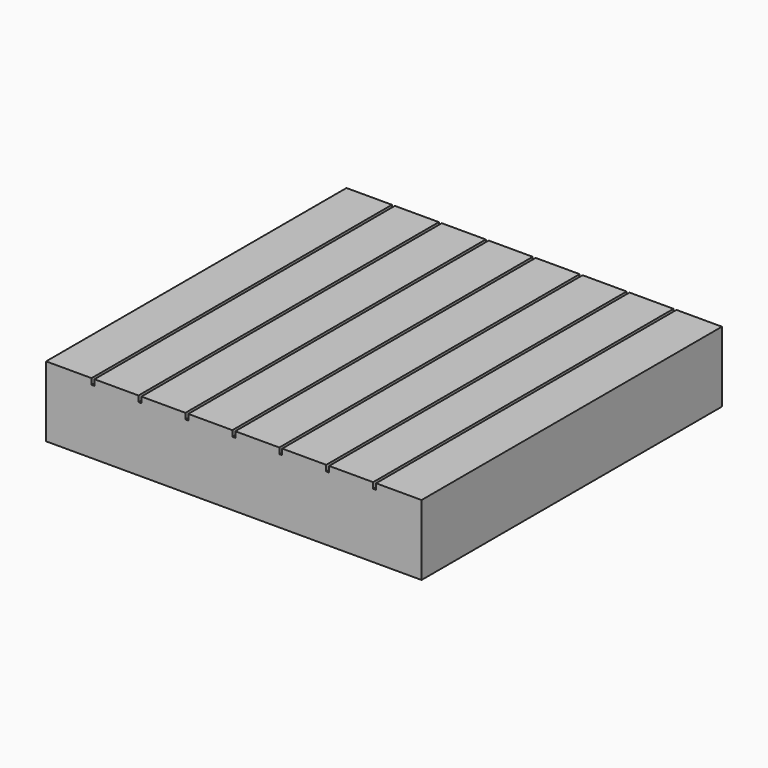
from build123d import *

# Parameters (mm, degrees)
F0_W     = 101.6
F0_H     = 101.6
F1_DEPTH = 19.05
F2_W     = 0.396875
F2_H     = 101.6
F3_DEPTH = 1.5875


# Not quite as in the source:
# - a length typed as a fraction of an inch, garbled in the dataset ("3 / 203.2 mm" for 3/8 in), is restored


with BuildPart() as f1:
    # F0 (on Top) → F1 (new body)
    with BuildSketch(Plane.XY):
        Rectangle(F0_W, F0_H)
    extrude(amount=F1_DEPTH)

    # F2 (on face) → F3 (cut)
    with BuildSketch(Plane.XY.offset(19.05)):
        with Locations((-38.2984375, 0)):
            Rectangle(F2_W, F2_H)
        with Locations((-37.9015625, 0)):
            Rectangle(F2_W, F2_H)
        with Locations((-25.5984375, 0)):
            Rectangle(F2_W, F2_H)
        with Locations((-25.2015625, 0)):
            Rectangle(F2_W, F2_H)
        with Locations((-12.8984375, 0)):
            Rectangle(F2_W, F2_H)
        with Locations((-12.5015625, 0)):
            Rectangle(F2_W, F2_H)
        with Locations((-0.1984375, 0)):
            Rectangle(F2_W, F2_H)
        with Locations((0.1984375, 0)):
            Rectangle(F2_W, F2_H)
        with Locations((12.5015625, 0)):
            Rectangle(F2_W, F2_H)
        with Locations((12.8984375, 0)):
            Rectangle(F2_W, F2_H)
        with Locations((25.2015625, 0)):
            Rectangle(F2_W, F2_H)
        with Locations((25.5984375, 0)):
            Rectangle(F2_W, F2_H)
        with Locations((37.9015625, 0)):
            Rectangle(F2_W, F2_H)
        with Locations((38.2984375, 0)):
            Rectangle(F2_W, F2_H)
    extrude(amount=-F3_DEPTH, mode=Mode.SUBTRACT)


solid = f1.part
